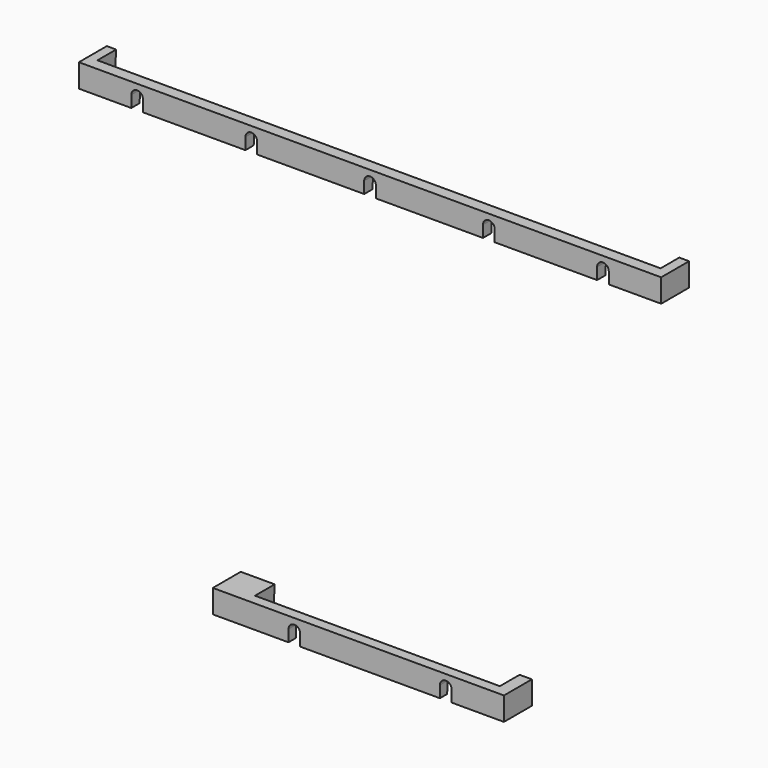
from build123d import *

# Parameters (mm, degrees)
F0_W     = 12.7
F0_H     = 25.4
F1_DEPTH = 38.1
F2_W     = 614.1419559717
F2_H     = 25.4462901503
F3_DEPTH = 25.4
F3_TAPER = -3
F4_W     = 267.035773024
F4_H     = 26.885855943
F5_DEPTH = 25.4
F5_TAPER = -3
F6_DEPTH = 25.4


# Not quite as in the source:
# - a feature of the source that left no trace in its solid (it failed there, or was rolled back) is left out


with BuildPart() as f1:
    # F0 (on Front) → F1 (new body)
    with BuildSketch(Plane.XZ):
        with Locations((204.3829661512, 207.5833906111)):
            Rectangle(F0_W, F0_H)
        with BuildLine():
            ThreePointArc((-367.1170338488, 207.5833906111), (-360.7670338488, 213.9333906111), (-354.4170338488, 207.5833906111))
            Line((-354.4170338488, 207.5833906111), (-354.4170338488, 194.8833906111))
            Line((-354.4170338488, 194.8833906111), (-242.6570338488, 194.8833906111))
            Line((-242.6570338488, 194.8833906111), (-242.6570338488, 207.5833906111))
            ThreePointArc((-242.6570338488, 207.5833906111), (-236.3070338488, 213.9333906111), (-229.9570338488, 207.5833906111))
            Line((-229.9570338488, 207.5833906111), (-229.9570338488, 194.8833906111))
            Line((-229.9570338488, 194.8833906111), (-113.1170338488, 194.8833906111))
            Line((-113.1170338488, 194.8833906111), (-113.1170338488, 207.5833906111))
            ThreePointArc((-113.1170338488, 207.5833906111), (-106.7670338488, 213.9333906111), (-100.4170338488, 207.5833906111))
            Line((-100.4170338488, 207.5833906111), (-100.4170338488, 194.8833906111))
            Line((-100.4170338488, 194.8833906111), (16.4229661512, 194.8833906111))
            Line((16.4229661512, 194.8833906111), (16.4229661512, 207.5833906111))
            ThreePointArc((16.4229661512, 207.5833906111), (22.7729661512, 213.9333906111), (29.1229661512, 207.5833906111))
            Line((29.1229661512, 207.5833906111), (29.1229661512, 194.8833906111))
            Line((29.1229661512, 194.8833906111), (140.8829827985, 194.8833906111))
            Line((140.8829827985, 194.8833906111), (140.8829827985, 207.5543100772))
            ThreePointArc((140.8829827985, 207.5543100772), (140.8829661512, 207.5688503442), (140.8829827985, 207.5833906112))
            ThreePointArc((140.8829827985, 207.5833906112), (147.2329661512, 213.9188503442), (153.582949504, 207.5833906111))
            ThreePointArc((153.582949504, 207.5833906111), (153.5829661512, 207.5688503442), (153.582949504, 207.5543100772))
            Line((153.582949504, 207.5543100772), (153.582949504, 194.8833906111))
            Line((153.582949504, 194.8833906111), (198.0329661512, 194.8833906111))
            Line((198.0329661512, 194.8833906111), (198.0329661512, 220.2833906111))
            Line((198.0329661512, 220.2833906111), (-411.5670338488, 220.2833906111))
            Line((-411.5670338488, 220.2833906111), (-424.2670338488, 220.2833906111))
            Line((-424.2670338488, 220.2833906111), (-424.2670338488, 194.8833906111))
            Line((-424.2670338488, 194.8833906111), (-411.5670338488, 194.8833906111))
            Line((-411.5670338488, 194.8833906111), (-367.1170338488, 194.8833906111))
            Line((-367.1170338488, 194.8833906111), (-367.1170338488, 207.5833906111))
        make_face()
    extrude(amount=F1_DEPTH)

    # F2 (on face) → F3 (cut)
    with BuildSketch(Plane.XY.offset(220.2833906111)):
        with Locations((-107.0529446006, -12.7231450751)):
            Rectangle(F2_W, F2_H)
    extrude(amount=-F3_DEPTH, taper=F3_TAPER, mode=Mode.SUBTRACT)


with BuildPart() as f1b:
    # F0 (on Front) → F1, piece 2 (new body)
    with BuildSketch(Plane.XZ):
        with BuildLine():
            ThreePointArc((-195.6670338488, -249.6166093889), (-189.3170338488, -243.2666093889), (-182.9670338488, -249.6166093889))
            Line((-182.9670338488, -249.6166093889), (-182.9670338488, -262.3166093889))
            Line((-182.9670338488, -262.3166093889), (-30.5670338488, -262.3166093889))
            Line((-30.5670338488, -262.3166093889), (-30.5670338488, -249.6166093889))
            ThreePointArc((-30.5670338488, -249.6166093889), (-24.2170338488, -243.2666093889), (-17.8670338488, -249.6166093889))
            Line((-17.8670338488, -249.6166093889), (-17.8670338488, -262.3166093889))
            Line((-17.8670338488, -262.3166093889), (39.2829661512, -262.3166093889))
            Line((39.2829661512, -262.3166093889), (39.2829661512, -236.9166093889))
            Line((39.2829661512, -236.9166093889), (-252.8170338488, -236.9166093889))
            Line((-252.8170338488, -236.9166093889), (-252.8170338488, -262.3166093889))
            Line((-252.8170338488, -262.3166093889), (-195.6670338488, -262.3166093889))
            Line((-195.6670338488, -262.3166093889), (-195.6670338488, -249.6166093889))
        make_face()
    extrude(amount=F1_DEPTH)

    # F4 (on face) → F5 (cut)
    with BuildSketch(Plane.XY.offset(-236.9166093889)):
        with Locations((-107.6784180477, -13.4429279715)):
            Rectangle(F4_W, F4_H)
    extrude(amount=-F5_DEPTH, taper=F5_TAPER, mode=Mode.SUBTRACT)

    # F6 (add): a face of the model
    f6_faces = [f1b.faces().sort_by_distance(p)[0] for p in [
        (-252.8170338488, -19.05, -249.6166093889),
    ]]
    extrude(f6_faces, amount=F6_DEPTH)


solid = Compound([f1.part, f1b.part])
